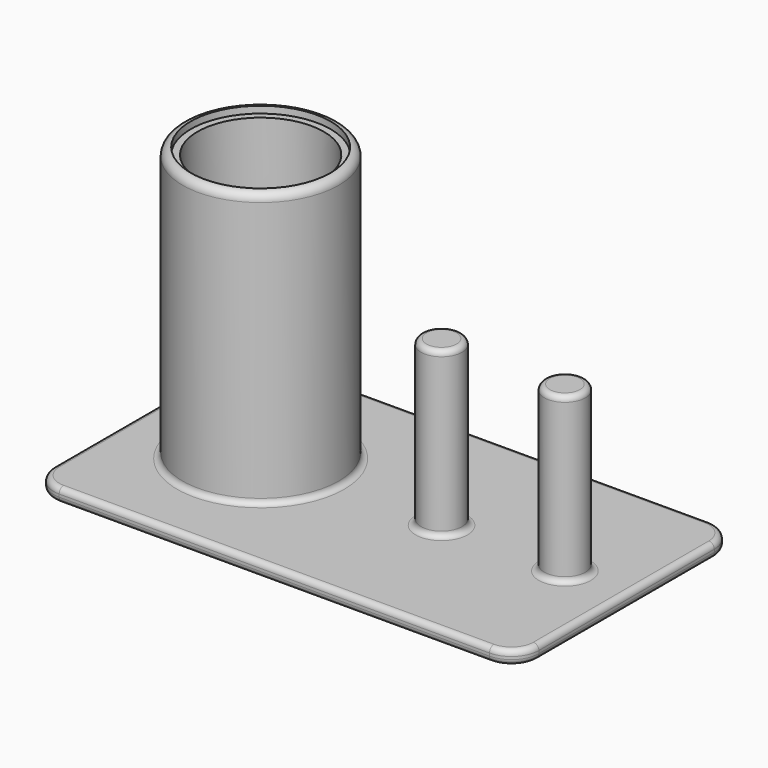
from build123d import *

# Parameters (mm, degrees)
F0_W     = 177
F0_H     = 100
F1_DEPTH = 5
F2_R     = 28.5
F3_DEPTH = 100
F4_R     = 10
F5_R     = 3
F6_DEPTH = 2.5
F7_R     = 23
F8_DEPTH = 27.5
F2_R_2   = 7.5
F9_DEPTH = 60
F10_R    = 2


# Not quite as in the source:
# - a feature names something its author has since deleted; it is built from what else it names


with BuildPart() as f1:
    # F0 (on Top) → F1 (new body)
    with BuildSketch(Plane.XY):
        with Locations((-34.2411024152, 50)):
            Rectangle(F0_W, F0_H)
    extrude(amount=F1_DEPTH)

    # F2 (on face) → F3 (join)
    with BuildSketch(Plane.XY.offset(5)):
        with Locations((-79.2411024152, 50)):
            Circle(F2_R)
    extrude(amount=F3_DEPTH)

    # F4
    f4_edges = [f1.edges().sort_by_distance(p)[0] for p in [
        (-122.741102, 0, 2.5),
        (54.258898, 0, 2.5),
        (-122.741102, 100, 2.5),
        (54.258898, 100, 2.5),
    ]]
    fillet(f4_edges, radius=F4_R)

    # F5
    f5_edges = [f1.edges().sort_by_distance(p)[0] for p in [
        (-107.741102, 50, 105),
    ]]
    fillet(f5_edges, radius=F5_R)

    # F6 (cut): a face of the model
    f6_faces = [f1.faces().sort_by_distance(p)[0] for p in [
        (-79.2411024152, 50, 105),
    ]]
    extrude(f6_faces, amount=-F6_DEPTH, mode=Mode.SUBTRACT)

    # F7 (on face) → F8 (cut)
    with BuildSketch(Plane.XY.offset(102.5)):
        with Locations((-79.2411024152, 50)):
            Circle(F7_R)
    extrude(amount=-F8_DEPTH, mode=Mode.SUBTRACT)

    # F2 (on face) → F9 (join)
    with BuildSketch(Plane.XY.offset(5)):
        with Locations((31.7588975848, 50)):
            Circle(F2_R_2)
        with Locations((-13.2411024152, 50)):
            Circle(F2_R_2)
    extrude(amount=F9_DEPTH)

    # F10
    f10_edges = [f1.edges().sort_by_distance(p)[0] for p in [
        (-34.241102, 0, 5),
        (-119.81217, 2.928932, 5),
        (51.329965, 2.928932, 5),
        (-122.741102, 50, 5),
        (54.258898, 50, 5),
        (-119.81217, 97.071068, 5),
        (51.329965, 97.071068, 5),
        (-34.241102, 100, 5),
        (-107.741102, 50, 5),
        (-20.741102, 50, 5),
        (24.258898, 50, 5),
        (-34.241102, 0, 0),
        (-119.81217, 2.928932, 0),
        (51.329965, 2.928932, 0),
        (-122.741102, 50, 0),
        (54.258898, 50, 0),
        (-119.81217, 97.071068, 0),
        (51.329965, 97.071068, 0),
        (-34.241102, 100, 0),
        (-102.241102, 50, 75),
        (24.258898, 50, 65),
        (-20.741102, 50, 65),
    ]]
    fillet(f10_edges, radius=F10_R)


solid = f1.part
